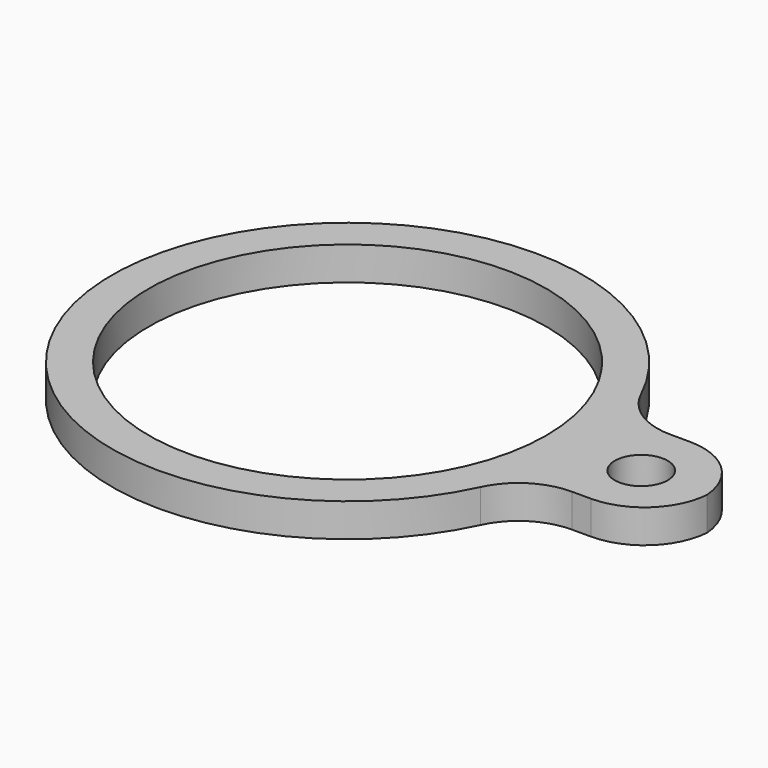
from build123d import *

# Parameters (mm, degrees)
F0_R        = 15.113
F0_R_2      = 2.0114491118
F1_DEPTH    = 2.54
F2_T1_DEPTH = 2.54
F2_T3_DEPTH = 27.94


# Not quite as in the source:
# - a fillet or chamfer that OpenCascade refuses, or shapes differently, is made with other operations: its cross-section is extruded or revolved along the edge and cut away or added


with BuildPart() as f1:
    # F0 (on Top) → F1 (new body)
    with BuildSketch(Plane.XY):
        with BuildLine():
            Line((27.3455847055, 4.693207435), (17.2810431679, 4.693207435))
            ThreePointArc((17.2810431679, 4.693207435), (-17.907, 0), (17.2810431679, -4.693207435))
            Line((17.2810431679, -4.693207435), (27.3455847055, -4.693207435))
            Line((27.3455847055, -4.693207435), (27.3455847055, 4.693207435))
        make_face()
        Circle(F0_R, mode=Mode.SUBTRACT)
        with Locations((22.3272647709, 0)):
            Circle(F0_R_2, mode=Mode.SUBTRACT)
    extrude(amount=F1_DEPTH)

    # F2: fillet of radius 5.08 on 4 edges, made by hand

    # F2_s2 → F2_t1 (join)
    with BuildSketch(Plane.XY):
        with BuildLine():
            ThreePointArc((16.2079318414, 7.6133825875), (18.0824647595, 5.4849496171), (20.8059266901, 4.693207435))
            Line((20.8059266901, 4.693207435), (17.2810431679, 4.693207435))
            ThreePointArc((17.2810431679, 4.693207435), (16.8080253904, 6.1766440301), (16.2079318414, 7.6133825875))
        make_face()
        with BuildLine():
            ThreePointArc((16.2079318414, -7.6133825875), (18.0824647595, -5.4849496171), (20.8059266901, -4.693207435))
            Line((20.8059266901, -4.693207435), (17.2810431679, -4.693207435))
            ThreePointArc((17.2810431679, -4.693207435), (16.8080253904, -6.1766440301), (16.2079318414, -7.6133825875))
        make_face()
    extrude(amount=F2_T1_DEPTH)

    # F2_s4 → F2_t3 (cut)
    with BuildSketch(Plane.XY.offset(-12.7)):
        with BuildLine():
            ThreePointArc((22.2655847055, -4.693207435), (25.8576871539, -3.2053098834), (27.3455847055, 0.386792565))
            Line((27.3455847055, 0.386792565), (27.3455847055, -4.693207435))
            Line((27.3455847055, -4.693207435), (22.2655847055, -4.693207435))
        make_face()
        with BuildLine():
            ThreePointArc((27.3455847055, -0.386792565), (25.8576871539, 3.2053098834), (22.2655847055, 4.693207435))
            Line((22.2655847055, 4.693207435), (27.3455847055, 4.693207435))
            Line((27.3455847055, 4.693207435), (27.3455847055, -0.386792565))
        make_face()
    extrude(amount=F2_T3_DEPTH, mode=Mode.SUBTRACT)


solid = f1.part
